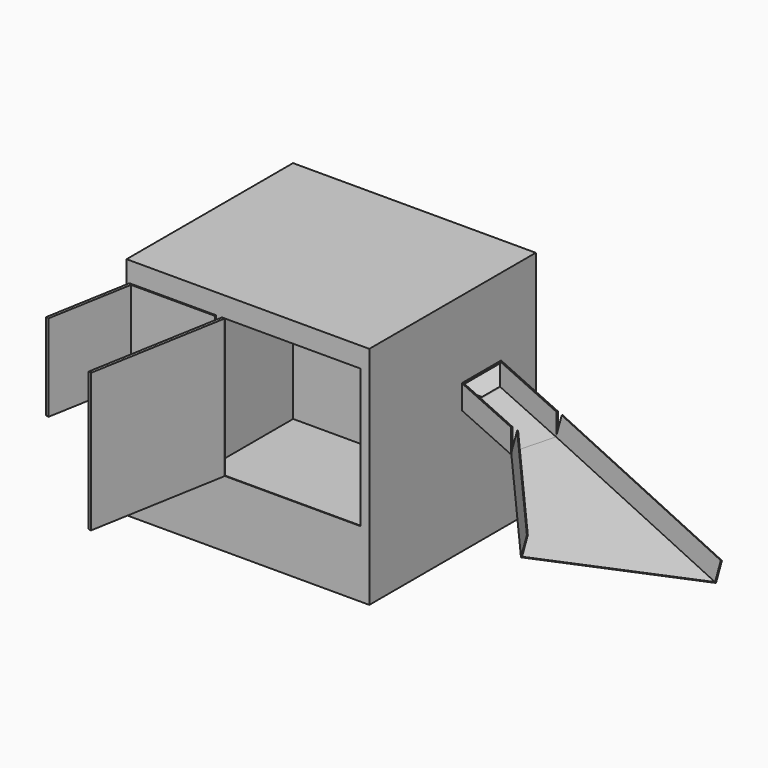
from build123d import *

# Parameters (mm, degrees)
F1_DEPTH    = 1981.2
F3_DEPTH    = 2184.401
F4_W        = 355.6
F4_H        = 901.7
F5_DEPTH    = 2717.801
F6_T        = 6.35
F6_T3_DEPTH = 381
F6_T5_DEPTH = 1536.7
F6_T7_DEPTH = 223.3713712335
F6_T9_DEPTH = 444.5
F8_DEPTH    = 196.85
F10_DEPTH   = 19.05
F11_W       = 762
F11_H       = 762
F11_W_2     = 1219.2
F11_H_2     = 1219.2
F12_DEPTH   = 12.7
F14_DEPTH   = 1219.2
F15_DEPTH   = 25.4
F17_DEPTH   = 762
F18_W       = 304.8
F18_H       = 304.8
F19_DEPTH   = 25.4
F20_W       = 101.6
F20_H       = 127
F20_R       = 19.05
F21_DEPTH   = 25.4
F23_DEPTH   = 196.85
F24_T       = -6.35


# Not quite as in the source:
# - a shell that OpenCascade refuses in one call is made with other operations: the cavity is built on its own and cut out


with BuildPart() as f1:
    # F0 (on Top) → F1 (new body)
    with BuildSketch(Plane.XY):
        Polygon((304.8, 1828.8), (0, 1828.8), (0, 0), (2133.6, 0), (2133.6, 1016), (2133.6, 1447.8), (2133.6, 1828.8), (1828.8, 1828.8), (1828.8, 2184.4), (304.8, 2184.4), align=None)
        Polygon((2133.6, 1447.8), (2133.6, 1016), (2641.6, 923.3724416764), (2717.8, 1341.2783079278), align=None)
    extrude(amount=F1_DEPTH)

    # F2 (on Front) → F3 (cut, through all)
    with BuildSketch(Plane.XZ):
        Polygon((2717.8, 1981.2), (2133.6, 1981.2), (2133.6, 1302.8713712335), (2717.8, 1143), align=None)
        Polygon((2133.6, 1092.2), (2133.6, 0), (2717.8, 0), (2717.8, 932.3286287665), align=None)
    extrude(amount=-F3_DEPTH, mode=Mode.SUBTRACT)

    # F4 (on face) → F5 (cut, through all)
    with BuildSketch(Plane(origin=(0, 0, 0), x_dir=(0, -1, 0), z_dir=(-1, 0, 0))):
        with Locations((-2006.6, 1530.35)):
            Rectangle(F4_W, F4_H)
        Polygon((-2184.4, 0), (-1828.8, 0), (-1828.8, 711.2), (-2184.4, 800.1), align=None)
    extrude(amount=-F5_DEPTH, mode=Mode.SUBTRACT)

    # F6: shell of thickness 6.35, made by hand


with BuildPart() as f6_core1:
    # F6_t2: copy of F1
    add(f1.part)

    # the walls: a layer under each face that stays
    f6_faces = [f6_core1.faces().sort_by_distance(p)[0] for p in [
        (1778, 1828.8, 1651),
        (1066.8, 2006.6, 755.65),
        (1066.8, 2184.4, 939.8),
        (1828.8, 2006.6, 895.35),
        (304.8, 2006.6, 895.35),
        (0, 914.4, 990.6),
        (1066.8, 0, 990.6),
        (1066.8, 914.4, 1981.2),
        (2133.6, 914.4, 990.6),
        (2425.7, 1185.5862208382, 1012.2643143833),
        (2679.7, 1132.3253748021, 1048.0907081594),
        (2387.6, 969.6862208382, 1128.0263937761),
        (2425.7, 1185.5862208382, 1222.9356856167),
        (2425.7, 1394.5391539639, 1117.6),
        (1066.8, 914.4, 0),
    ]]
    thicken(f6_faces, amount=-F6_T, mode=Mode.SUBTRACT)

    # F6_s4 → F6_t3 (cut)
    with BuildSketch(Plane.XY.offset(704.85)):
        Polygon((304.7365, 1828.8635), (304.8, 1822.45), (311.15, 1822.45), (311.15, 1828.8), align=None)
        Polygon((1828.8635, 1828.8635), (1828.8, 1822.45), (1822.45, 1822.45), (1822.45, 1828.8), align=None)
    extrude(amount=F6_T3_DEPTH, mode=Mode.SUBTRACT)

    # F6_s6 → F6_t5 (cut)
    with BuildSketch(Plane.YZ.offset(298.45)):
        Polygon((1828.8789010122, 711.1383959512), (1822.45, 711.2), (1822.45, 716.1579301807), (1827.259898781, 717.3604048759), align=None)
    extrude(amount=F6_T5_DEPTH, mode=Mode.SUBTRACT)

    # F6_s8 → F6_t7 (cut)
    with BuildSketch(Plane.XY.offset(1085.85)):
        Polygon((2133.6748906405, 1447.8624700193), (2127.25, 1447.8), (2127.25, 1442.5031482168), (2132.4609359537, 1441.5529980712), align=None)
        Polygon((2133.6521093595, 1015.9375299807), (2127.25, 1016), (2127.25, 1023.6125407413), (2134.7390640463, 1022.2470019288), align=None)
    extrude(amount=F6_T7_DEPTH, mode=Mode.SUBTRACT)

    # F6_s10 → F6_t9 (cut)
    with BuildSketch(Plane.XZ.offset(-1454.15)):
        Polygon((2133.6802610435, 1302.9326192328), (2127.25, 1302.8713712335), (2127.25, 1298.0256231785), (2131.9238956462, 1296.7465713025), align=None)
        Polygon((2133.6467389565, 1092.1387520007), (2127.25, 1092.2), (2127.25, 1100.5212126471), (2135.2761043538, 1098.324799931), align=None)
    extrude(amount=F6_T9_DEPTH, mode=Mode.SUBTRACT)


with BuildPart() as f1_1:
    add(f1.part)

    # what is left inside the walls is the cavity
    f6_cavity = [f6_core1.part.solids().sort_by_distance(p)[0] for p in [
        (1066.8, 6.4135, 1318.683333),
    ]]
    add(f6_cavity, mode=Mode.SUBTRACT)

    # F7 (on face) → F8 (cut)
    with BuildSketch(Plane(origin=(480.3521470905, 0, 1755.2969125438), x_dir=(0.9645354222, 0, -0.2639534415), z_dir=(0.2639534415, 0, 0.9645354222))):
        Polygon((1726.7353944944, 1026.6613500194), (2230.5640168439, 938.0524140666), (2304.8472958363, 1330.9982978041), (1726.7353944944, 1432.6715219268), align=None)
    extrude(amount=-F8_DEPTH, mode=Mode.SUBTRACT)

    # F9 (on face) → F10 (cut)
    with BuildSketch(Plane(origin=(2393.6525155954, -436.4531259741, 0), x_dir=(0.1793801648, 0.9837798313, 0), z_dir=(0.9837798313, -0.1793801648, 0))):
        Polygon((1794.3562029508, 945.6666515071), (1794.3562029508, 1143.6227302064), (1394.9315845226, 1163.2300573458), (1394.9315845226, 965.2739786465), align=None)
        Polygon((1394.9315845226, 1163.2300573458), (1794.3562029508, 1143.6227302064), (1798.9468574524, 1186.6028308868), (1379.6262741089, 1213.9142751694), align=None)
    extrude(amount=-F10_DEPTH, mode=Mode.SUBTRACT)

    # F11 (on face) → F12 (join)
    with BuildSketch(Plane.XZ):
        with Locations((406.4, 1422.4)):
            Rectangle(F11_W, F11_H)
        with Locations((1447.8, 1193.8)):
            Rectangle(F11_W_2, F11_H_2)
    extrude(amount=F12_DEPTH)

    # F13 (on face) → F14 (join, through all)
    with BuildSketch(Plane.XY.offset(1803.4)):
        with BuildLine():
            Line((838.2, 0), (626.4881417885, -1200.6776124725))
            ThreePointArc((626.4881417885, -1200.6776124725), (639.0073665936, -1202.8179142317), (651.548208115, -1204.8276841881))
            Line((651.548208115, -1204.8276841881), (861.7524832869, -12.7))
            Line((861.7524832869, -12.7), (838.2, -12.7))
            Line((838.2, -12.7), (838.2, 0))
        make_face()
    extrude(amount=-F14_DEPTH)

    # F15 (cut): a face of the model
    f15_faces = [f1_1.faces().sort_by_distance(p)[0] for p in [
        (1459.5762416435, -12.7, 1193.8),
    ]]
    extrude(f15_faces, amount=-F15_DEPTH, mode=Mode.SUBTRACT)

    # F16 (on face) → F17 (join, through all)
    with BuildSketch(Plane.XY.offset(1803.4)):
        with BuildLine():
            Line((25.4, 0), (-106.9199113822, -750.4235077953))
            ThreePointArc((-106.9199113822, -750.4235077953), (-94.3927308322, -752.524884399), (-81.8322629627, -754.4171536888))
            Line((-81.8322629627, -754.4171536888), (48.9524832869, -12.7))
            Line((48.9524832869, -12.7), (25.4, -12.7))
            Line((25.4, -12.7), (25.4, 0))
        make_face()
    extrude(amount=-F17_DEPTH)

    # F18 (on face) → F19 (join)
    with BuildSketch(Plane(origin=(0, 1828.8, 0), x_dir=(-1, 0, 0), z_dir=(0, 1, 0))):
        with Locations((-177.8, 1473.2)):
            Rectangle(F18_W, F18_H)
    extrude(amount=F19_DEPTH)

    # F20 (on face) → F21 (join)
    with BuildSketch(Plane(origin=(0, 1854.2, 0), x_dir=(-1, 0, 0), z_dir=(0, 1, 0))):
        with Locations((-228.6, 1511.3)):
            Rectangle(F20_W, F20_H)
        with Locations((-127, 1511.3)):
            Rectangle(F20_W, F20_H)
        with Locations((-215.9, 1371.6)):
            Circle(F20_R)
        with Locations((-139.7, 1371.6)):
            Circle(F20_R)
    extrude(amount=F21_DEPTH)


with BuildPart() as f23:
    # F22 (on face) → F23 (new body, through all)
    with BuildSketch(Plane(origin=(428.392912122, 0, 1565.428114682), x_dir=(0.9645354222, 0, -0.2639534415), z_dir=(0.2639534415, 0, 0.9645354222))):
        Polygon((2365.9276469879, 1336.1703700453), (2289.2877743556, 930.7585076514), (3086.5123505597, 76.5972025713), (4088.1940606272, 1011.5087609039), align=None)
    extrude(amount=F23_DEPTH)

    # F24
    f24_openings = [f23.faces().sort_by_distance(p)[0] for p in [
        (3451.053503, 803.590618, 942.338851),
        (3914.501768, 544.052982, 713.468289),
        (2699.432616, 1133.464439, 1045.982448),
    ]]
    offset(amount=F24_T, openings=f24_openings)


solid = Compound([f1_1.part, f23.part])
